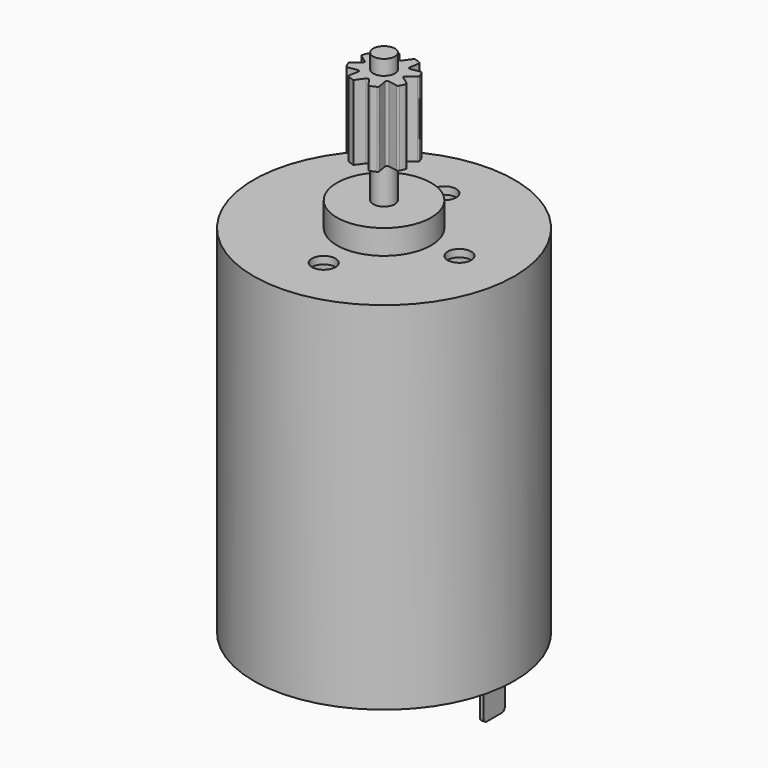
from build123d import *

# Parameters (mm, degrees)
F0_R         = 13.85
F1_DEPTH     = 37.8
F2_R         = 5
F3_DEPTH     = 2.6
F4_R         = 1.25
F5_DEPTH     = 0.79375
F6_R         = 13.05625
F7_DEPTH     = 37.0062506
F8_R         = 1.15
F9_DEPTH     = 50.8
F11_R        = 13.05625
F12_DEPTH    = 0.79375
F13_R        = 5
F14_DEPTH    = 2.6
F15_R        = 1.15
F16_DEPTH    = 25.4
F10_R        = 1.15
F17_DEPTH    = 13.8
F18_DEPTH    = 43.2
F19_W        = 0.4
F19_H        = 2.8
F20_DEPTH    = 4.1
F21_R        = 0.396875
F21_2_R      = 0.396875
F22_R        = 3.175
F22_R_2      = 1.15
F23_DEPTH    = 9.525
F24_DEPTH    = 1.5875
F26_DEPTH    = 25.4
F27_R        = 0.1984375
F28_T1_DEPTH = 8.6642936454


# Not quite as in the source:
# - a fillet or chamfer that OpenCascade refuses, or shapes differently, is made with other operations: its cross-section is extruded or revolved along the edge and cut away or added


with BuildPart() as f1:
    # F0 (on Top) → F1 (new body)
    with BuildSketch(Plane.XY):
        Circle(F0_R)
    extrude(amount=F1_DEPTH)

    # F2 (on face) → F3 (join)
    with BuildSketch(Plane.XY.offset(37.8)):
        Circle(F2_R)
    extrude(amount=F3_DEPTH)

    # F4 (on face) → F5 (cut)
    with BuildSketch(Plane.XY.offset(37.8)):
        with Locations((0, 8)):
            Circle(F4_R)
        with Locations((8, 0)):
            Circle(F4_R)
        with Locations((0, -8)):
            Circle(F4_R)
    extrude(amount=-F5_DEPTH, mode=Mode.SUBTRACT)

    # F6 (on face) → F7 (cut)
    with BuildSketch(Plane(origin=(0, 0, 0), x_dir=(1, 0, 0), z_dir=(0, 0, -1))):
        Circle(F6_R)
    extrude(amount=-F7_DEPTH, mode=Mode.SUBTRACT)

    # F8 (on face) → F9 (cut)
    with BuildSketch(Plane.XY.offset(40.4)):
        Circle(F8_R)
    extrude(amount=-F9_DEPTH, mode=Mode.SUBTRACT)

    # F11 (on face) → F12 (join)
    with BuildSketch(Plane(origin=(0, 0, 0), x_dir=(1, 0, 0), z_dir=(0, 0, -1))):
        Circle(F11_R)
    extrude(amount=-F12_DEPTH)

    # F13 (on face) → F14 (join)
    with BuildSketch(Plane(origin=(0, 0, 0), x_dir=(1, 0, 0), z_dir=(0, 0, -1))):
        Circle(F13_R)
    extrude(amount=F14_DEPTH)

    # F15 (on face) → F16 (cut)
    with BuildSketch(Plane(origin=(0, 0, -2.6), x_dir=(1, 0, 0), z_dir=(0, 0, -1))):
        Circle(F15_R)
    extrude(amount=-F16_DEPTH, mode=Mode.SUBTRACT)


with BuildPart() as f17:
    # F10 (on face) → F17 (new body)
    with BuildSketch(Plane.XY.offset(40.4)):
        Circle(F10_R)
    extrude(amount=F17_DEPTH)

    # F18 (add): a face of the model
    f18_faces = [f17.faces().sort_by_distance(p)[0] for p in [
        (0, 0, 40.4),
    ]]
    extrude(f18_faces, amount=F18_DEPTH)


with BuildPart() as f20:
    # F19 (on face) → F20 (new body)
    with BuildSketch(Plane(origin=(0, 0, 0), x_dir=(1, 0, 0), z_dir=(0, 0, -1))):
        with Locations((-11.5, 0)):
            Rectangle(F19_W, F19_H)
    extrude(amount=F20_DEPTH)

    # F21
    f21_edges = [f20.edges().sort_by_distance(p)[0] for p in [
        (-11.5, 1.4, -4.1),
        (-11.5, -1.4, -4.1),
    ]]
    fillet(f21_edges, radius=F21_R)


with BuildPart() as f20b:
    # F19 (on face) → F20, piece 2 (new body)
    with BuildSketch(Plane(origin=(0, 0, 0), x_dir=(1, 0, 0), z_dir=(0, 0, -1))):
        with Locations((11.5, 0)):
            Rectangle(F19_W, F19_H)
    extrude(amount=F20_DEPTH)

    # F21#2
    f21_2_edges = [f20b.edges().sort_by_distance(p)[0] for p in [
        (11.5, -1.4, -4.1),
        (11.5, 1.4, -4.1),
    ]]
    fillet(f21_2_edges, radius=F21_2_R)


with BuildPart() as f23:
    # F22 (on face) → F23 (new body)
    with BuildSketch(Plane.XY.offset(54.2)):
        Circle(F22_R)
        Circle(F22_R_2, mode=Mode.SUBTRACT)
    extrude(amount=-F23_DEPTH)

    # F24 (cut): a face of the model
    f24_faces = [f23.faces().sort_by_distance(p)[0] for p in [
        (-3.0851974388, 0, 54.2),
    ]]
    extrude(f24_faces, amount=-F24_DEPTH, mode=Mode.SUBTRACT)

    # F25 (on face) → F26 (cut)
    with BuildSketch(Plane.XY.offset(52.6125)):
        with BuildLine():
            ThreePointArc((-1.6125078925, 2.7350399077), (-2.2450640303, 2.2450640303), (-2.7350399077, 1.6125078925))
            Line((-2.7350399077, 1.6125078925), (-1.3744388059, 1.3744388059))
            Line((-1.3744388059, 1.3744388059), (-1.6125078925, 2.7350399077))
        make_face()
        with BuildLine():
            ThreePointArc((0.79375, 3.0741805311), (0, 3.175), (-0.79375, 3.0741805311))
            Line((-0.79375, 3.0741805311), (0, 1.94375))
            Line((0, 1.94375), (0.79375, 3.0741805311))
        make_face()
        with BuildLine():
            ThreePointArc((2.7350399077, 1.6125078925), (2.2450640303, 2.2450640303), (1.6125078925, 2.7350399077))
            Line((1.6125078925, 2.7350399077), (1.3744388059, 1.3744388059))
            Line((1.3744388059, 1.3744388059), (2.7350399077, 1.6125078925))
        make_face()
        with BuildLine():
            ThreePointArc((3.175, 0), (3.1496942856, 0.4000636286), (3.0741805311, 0.79375))
            Line((3.0741805311, 0.79375), (1.94375, 0))
            Line((1.94375, 0), (3.0741805311, -0.79375))
            ThreePointArc((3.0741805311, -0.79375), (3.1496942856, -0.4000636286), (3.175, 0))
        make_face()
        with BuildLine():
            Line((1.3744388059, -1.3744388059), (1.6125078925, -2.7350399077))
            ThreePointArc((1.6125078925, -2.7350399077), (2.2450640303, -2.2450640303), (2.7350399077, -1.6125078925))
            Line((2.7350399077, -1.6125078925), (1.3744388059, -1.3744388059))
        make_face()
        with BuildLine():
            Line((0, -1.94375), (-0.79375, -3.0741805311))
            ThreePointArc((-0.79375, -3.0741805311), (0, -3.175), (0.79375, -3.0741805311))
            Line((0.79375, -3.0741805311), (0, -1.94375))
        make_face()
        with BuildLine():
            Line((-1.3744388059, -1.3744388059), (-2.7350399077, -1.6125078925))
            ThreePointArc((-2.7350399077, -1.6125078925), (-2.2450640303, -2.2450640303), (-1.6125078925, -2.7350399077))
            Line((-1.6125078925, -2.7350399077), (-1.3744388059, -1.3744388059))
        make_face()
        with BuildLine():
            Line((-3.0741805311, -0.79375), (-1.94375, 0))
            Line((-1.94375, 0), (-3.0741805311, 0.79375))
            ThreePointArc((-3.0741805311, 0.79375), (-3.175, 0), (-3.0741805311, -0.79375))
        make_face()
    extrude(amount=-F26_DEPTH, mode=Mode.SUBTRACT)

    # F27
    f27_edges = [f23.edges().sort_by_distance(p)[0] for p in [
        (-1.374439, 1.374439, 48.64375),
        (0, 1.94375, 48.64375),
        (1.374439, 1.374439, 48.64375),
        (1.94375, 0, 48.64375),
        (1.374439, -1.374439, 48.64375),
        (0, -1.94375, 48.64375),
        (-1.374439, -1.374439, 48.64375),
        (-1.94375, 0, 48.64375),
    ]]
    fillet(f27_edges, radius=F27_R)

    # F28: fillet of radius 0.1984375 on 15 edges, made by hand

    # F28_s2 → F28_t1 (cut)
    with BuildSketch(Plane.XY.offset(44.3116031773)):
        with BuildLine():
            add(Edge.make_bspline(
                [(-3.034628604, 0.9336242477), (-3.0770434151, 0.7957602201), (-2.9589967221, 0.7128718338)],
                knots=[0, 0, 0, 1, 1, 1], degree=2, weights=[1, 1, 1]))
            Line((-2.9589967221, 0.7128718338), (-3.0741805311, 0.79375))
            ThreePointArc((-3.0741805311, 0.79375), (-3.0552051426, 0.8639135007), (-3.034628604, 0.9336242477))
        make_face()
        with BuildLine():
            add(Edge.make_bspline(
                [(-3.034628604, -0.9336242477), (-3.0770434151, -0.7957602201), (-2.9589967221, -0.7128718338)],
                knots=[0, 0, 0, 1, 1, 1], degree=2, weights=[1, 1, 1]))
            Line((-2.9589967221, -0.7128718338), (-3.0741805311, -0.79375))
            ThreePointArc((-3.0741805311, -0.79375), (-3.0552051426, -0.8639135007), (-3.034628604, -0.9336242477))
        make_face()
        with BuildLine():
            add(Edge.make_bspline(
                [(-2.5964031555, -1.5882501399), (-2.7384857127, -1.613110817), (-2.8059785009, -1.4856344276)],
                knots=[0, 0, 0, 1, 1, 1], degree=2, weights=[1, 1, 1]))
            ThreePointArc((-2.8059785009, -1.4856344276), (-2.7712353689, -1.5494771795), (-2.7350399077, -1.6125078925))
            Line((-2.7350399077, -1.6125078925), (-2.5964031555, -1.5882501399))
        make_face()
        with BuildLine():
            add(Edge.make_bspline(
                [(-2.5964031555, 1.5882501399), (-2.7384857127, 1.613110817), (-2.8059785009, 1.4856344276)],
                knots=[0, 0, 0, 1, 1, 1], degree=2, weights=[1, 1, 1]))
            ThreePointArc((-2.8059785009, 1.4856344276), (-2.7712353689, 1.5494771795), (-2.7350399077, 1.6125078925))
            Line((-2.7350399077, 1.6125078925), (-2.5964031555, 1.5882501399))
        make_face()
        with BuildLine():
            add(Edge.make_bspline(
                [(-1.4856344276, 2.8059785009), (-1.613110817, 2.7384857127), (-1.5882501399, 2.5964031555)],
                knots=[0, 0, 0, 1, 1, 1], degree=2, weights=[1, 1, 1]))
            Line((-1.5882501399, 2.5964031555), (-1.6125078925, 2.7350399077))
            ThreePointArc((-1.6125078925, 2.7350399077), (-1.5494771795, 2.7712353689), (-1.4856344276, 2.8059785009))
        make_face()
        with BuildLine():
            add(Edge.make_bspline(
                [(-0.7128718338, 2.9589967221), (-0.7957602201, 3.0770434151), (-0.9336242477, 3.034628604)],
                knots=[0, 0, 0, 1, 1, 1], degree=2, weights=[1, 1, 1]))
            ThreePointArc((-0.9336242477, 3.034628604), (-0.8639135007, 3.0552051426), (-0.79375, 3.0741805311))
            Line((-0.79375, 3.0741805311), (-0.7128718338, 2.9589967221))
        make_face()
        with BuildLine():
            add(Edge.make_bspline(
                [(0.9336242477, 3.034628604), (0.7957602201, 3.0770434151), (0.7128718338, 2.9589967221)],
                knots=[0, 0, 0, 1, 1, 1], degree=2, weights=[1, 1, 1]))
            Line((0.7128718338, 2.9589967221), (0.79375, 3.0741805311))
            ThreePointArc((0.79375, 3.0741805311), (0.8639135007, 3.0552051426), (0.9336242477, 3.034628604))
        make_face()
        with BuildLine():
            add(Edge.make_bspline(
                [(1.5882501399, 2.5964031555), (1.613110817, 2.7384857127), (1.4856344276, 2.8059785009)],
                knots=[0, 0, 0, 1, 1, 1], degree=2, weights=[1, 1, 1]))
            ThreePointArc((1.4856344276, 2.8059785009), (1.5494771795, 2.7712353689), (1.6125078925, 2.7350399077))
            Line((1.6125078925, 2.7350399077), (1.5882501399, 2.5964031555))
        make_face()
        with BuildLine():
            add(Edge.make_bspline(
                [(2.8059785009, 1.4856344276), (2.7384857127, 1.613110817), (2.5964031555, 1.5882501399)],
                knots=[0, 0, 0, 1, 1, 1], degree=2, weights=[1, 1, 1]))
            Line((2.5964031555, 1.5882501399), (2.7350399077, 1.6125078925))
            ThreePointArc((2.7350399077, 1.6125078925), (2.7712353689, 1.5494771795), (2.8059785009, 1.4856344276))
        make_face()
        with BuildLine():
            add(Edge.make_bspline(
                [(2.9589967221, 0.7128718338), (3.0770434151, 0.7957602201), (3.034628604, 0.9336242477)],
                knots=[0, 0, 0, 1, 1, 1], degree=2, weights=[1, 1, 1]))
            ThreePointArc((3.034628604, 0.9336242477), (3.0552051426, 0.8639135007), (3.0741805311, 0.79375))
            Line((3.0741805311, 0.79375), (2.9589967221, 0.7128718338))
        make_face()
        with BuildLine():
            add(Edge.make_bspline(
                [(2.9589967221, -0.7128718338), (3.0770434151, -0.7957602201), (3.034628604, -0.9336242477)],
                knots=[0, 0, 0, 1, 1, 1], degree=2, weights=[1, 1, 1]))
            ThreePointArc((3.034628604, -0.9336242477), (3.0552051426, -0.8639135007), (3.0741805311, -0.79375))
            Line((3.0741805311, -0.79375), (2.9589967221, -0.7128718338))
        make_face()
        with BuildLine():
            add(Edge.make_bspline(
                [(2.8059785009, -1.4856344276), (2.7384857127, -1.613110817), (2.5964031555, -1.5882501399)],
                knots=[0, 0, 0, 1, 1, 1], degree=2, weights=[1, 1, 1]))
            Line((2.5964031555, -1.5882501399), (2.7350399077, -1.6125078925))
            ThreePointArc((2.7350399077, -1.6125078925), (2.7712353689, -1.5494771795), (2.8059785009, -1.4856344276))
        make_face()
        with BuildLine():
            add(Edge.make_bspline(
                [(1.5882501399, -2.5964031555), (1.613110817, -2.7384857127), (1.4856344276, -2.8059785009)],
                knots=[0, 0, 0, 1, 1, 1], degree=2, weights=[1, 1, 1]))
            ThreePointArc((1.4856344276, -2.8059785009), (1.5494771795, -2.7712353689), (1.6125078925, -2.7350399077))
            Line((1.6125078925, -2.7350399077), (1.5882501399, -2.5964031555))
        make_face()
        with BuildLine():
            add(Edge.make_bspline(
                [(0.9336242477, -3.034628604), (0.7957602201, -3.0770434151), (0.7128718338, -2.9589967221)],
                knots=[0, 0, 0, 1, 1, 1], degree=2, weights=[1, 1, 1]))
            Line((0.7128718338, -2.9589967221), (0.79375, -3.0741805311))
            ThreePointArc((0.79375, -3.0741805311), (0.8639135007, -3.0552051426), (0.9336242477, -3.034628604))
        make_face()
        with BuildLine():
            add(Edge.make_bspline(
                [(-1.4856344276, -2.8059785009), (-1.613110817, -2.7384857127), (-1.5882501399, -2.5964031555)],
                knots=[0, 0, 0, 1, 1, 1], degree=2, weights=[1, 1, 1]))
            Line((-1.5882501399, -2.5964031555), (-1.6125078925, -2.7350399077))
            ThreePointArc((-1.6125078925, -2.7350399077), (-1.5494771795, -2.7712353689), (-1.4856344276, -2.8059785009))
        make_face()
    extrude(amount=F28_T1_DEPTH, mode=Mode.SUBTRACT)


solid = Compound([f1.part, f17.part, f20.part, f20b.part, f23.part])
